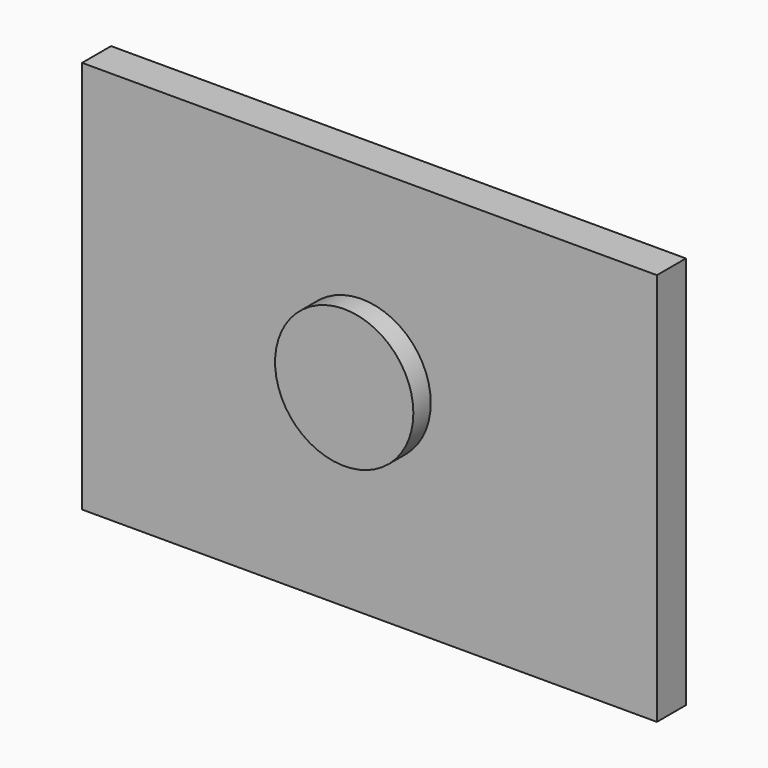
from build123d import *

# Parameters (mm, degrees)
F0_W     = 79.294
F0_H     = 54.2539670305
F1_DEPTH = 5
F2_R     = 9.5370045267
F3_DEPTH = 3


# Not quite as in the source:
# - the program builds the solid bodies; features that only make, move or delete a surface that nothing else refers to are left out


with BuildPart() as f1:
    # F0 (on Front) → F1 (new body)
    with BuildSketch(Plane.XZ):
        with Locations((1.0885317774, -1.4516480646)):
            Rectangle(F0_W, F0_H)
    extrude(amount=-F1_DEPTH)

    # F2 (on face) → F3 (join)
    with BuildSketch(Plane.XZ):
        Circle(F2_R)
    extrude(amount=F3_DEPTH)


solid = f1.part
